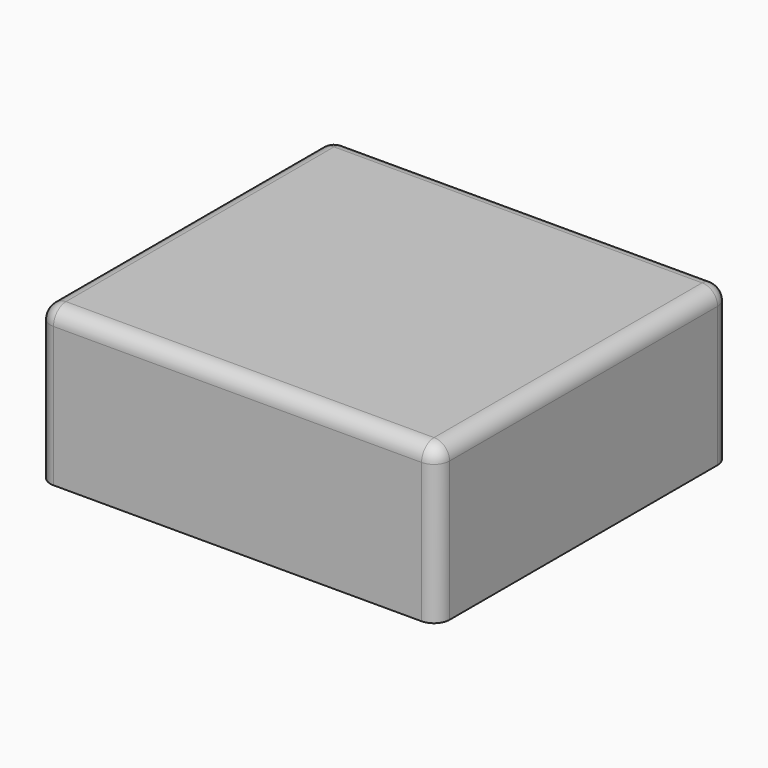
from build123d import *

# Parameters (mm, degrees)
F0_W     = 65.2412325144
F0_H     = 59.8419681191
F1_DEPTH = 25.4
F2_R     = 2.54
F3_T     = 2.54
F4_R     = 2.54


# Not quite as in the source:
# - a shell that OpenCascade refuses in one call is made with other operations: the cavity is built on its own and cut out


with BuildPart() as f1:
    # F0 (on Top) → F1 (new body)
    with BuildSketch(Plane.XY):
        with Locations((32.6206162572, 29.9209840596)):
            Rectangle(F0_W, F0_H)
    extrude(amount=F1_DEPTH)

    # F2
    f2_edges = [f1.edges().sort_by_distance(p)[0] for p in [
        (32.620616, 0, 25.4),
        (65.241233, 29.920984, 25.4),
        (32.620616, 59.841968, 25.4),
        (0, 29.920984, 25.4),
        (65.241233, 0, 12.7),
        (0, 0, 12.7),
        (65.241233, 59.841968, 12.7),
        (0, 59.841968, 12.7),
    ]]
    fillet(f2_edges, radius=F2_R)

    # F3: shell of thickness 2.54, made by hand


with BuildPart() as f3_core1:
    # F3_t2: copy of F1
    add(f1.part)

    # the walls: a layer under each face that stays
    f3_faces = [f3_core1.faces().sort_by_distance(p)[0] for p in [
        (0, 29.9209840596, 11.43),
        (32.6206162572, 59.8419681191, 11.43),
        (32.6206162572, 0, 11.43),
        (65.2412325144, 29.9209840596, 11.43),
        (32.6206162572, 29.9209840596, 25.4),
    ]]
    thicken(f3_faces, amount=-F3_T, mode=Mode.SUBTRACT)


with BuildPart() as f1_1:
    add(f1.part)

    # what is left inside the walls is the cavity
    f3_cavity = [f3_core1.part.solids().sort_by_distance(p)[0] for p in [
        (32.620616, 20.793989, 0.0254),
    ]]
    add(f3_cavity, mode=Mode.SUBTRACT)

    # F4
    f4_edges = [f1_1.edges().sort_by_distance(p)[0] for p in [
        (32.620616, 2.54, 22.86),
        (2.54, 29.920984, 22.86),
        (62.701233, 29.920984, 22.86),
        (32.620616, 57.301968, 22.86),
        (62.701233, 57.301968, 11.43),
        (2.54, 57.301968, 11.43),
        (2.54, 2.54, 11.43),
        (62.701233, 2.54, 11.43),
    ]]
    fillet(f4_edges, radius=F4_R)


solid = f1_1.part
